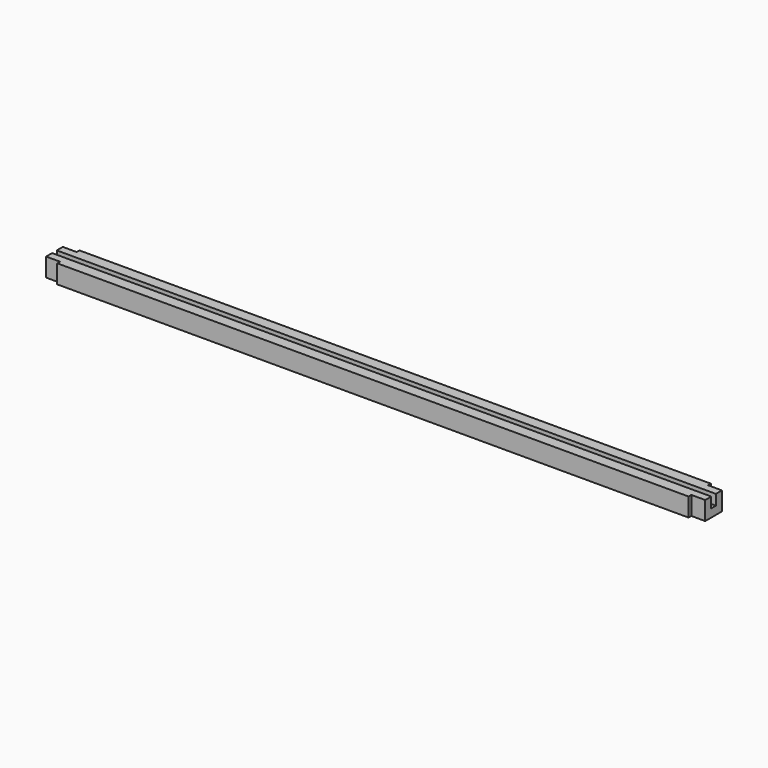
from build123d import *

# Parameters (mm, degrees)
F0_W     = 19.05
F0_H     = 12.7
F1_DEPTH = 225.425
F2_W     = 3.96875
F2_H     = 7.14375
F3_DEPTH = 450.85
F4_W     = 9.525
F4_H     = 2.38125
F5_DEPTH = 12.7


# Not quite as in the source:
# - a pattern or mirror of a feature is missing from the dataset's text; its kind, count and spacing are read off the source's solid


with BuildPart() as f1:
    # F0 (on Right) → F1 (new body, symmetric)
    with BuildSketch(Plane.YZ):
        with Locations((9.525, 6.35)):
            Rectangle(F0_W, F0_H)
    extrude(amount=F1_DEPTH, both=True)

    # F2 (on face) → F3 (cut, through all)
    with BuildSketch(Plane.YZ.offset(225.425)):
        with Locations((9.525, 9.128125)):
            Rectangle(F2_W, F2_H)
    extrude(amount=-F3_DEPTH, mode=Mode.SUBTRACT)

    # F4 (on face) → F5 (cut, through all)
    with BuildSketch(Plane.XY.offset(12.7)):
        with Locations((220.6625, 17.859375)):
            Rectangle(F4_W, F4_H)
        with Locations((220.6625, 1.190625)):
            Rectangle(F4_W, F4_H)
    f5 = extrude(amount=-F5_DEPTH, mode=Mode.SUBTRACT)

    # F5_copies: F5 across plane
    add(f5.mirror(Plane(origin=(0, 0, 0), x_dir=(0, 0, -1), z_dir=(-1, 0, 0))), mode=Mode.SUBTRACT)


solid = f1.part
